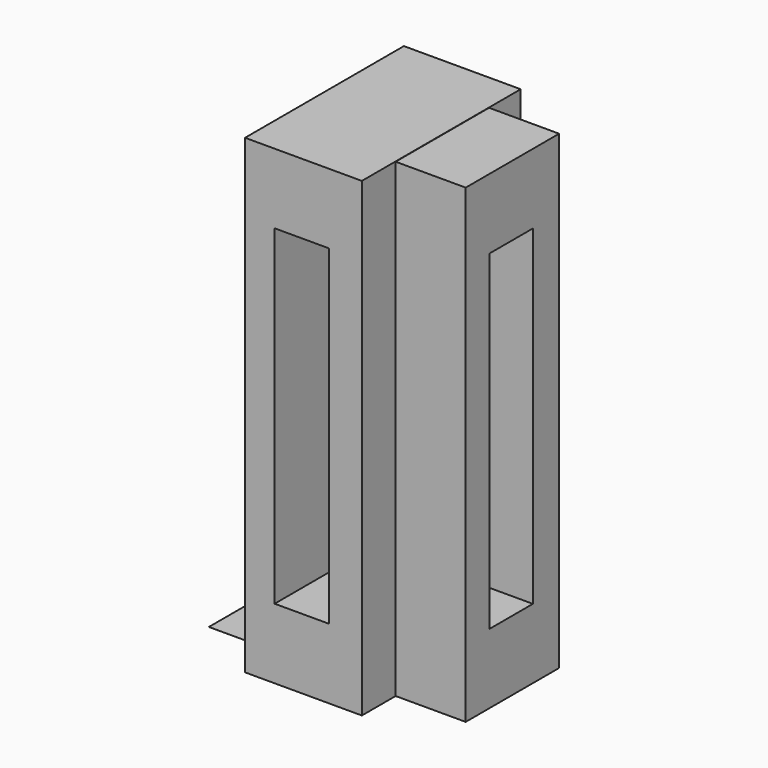
from build123d import *

# Parameters (mm, degrees)
F0_W     = 10
F0_H     = 40.3
F0_W_2   = 4.6593984449
F0_H_2   = 28.3
F1_DEPTH = 8.5
F2_DEPTH = 7
F4_W     = 10
F4_H     = 0.0023088843
F5_DEPTH = 6
F4_W_2   = 4.6593984449
F4_H_2   = 28.3
F6_DEPTH = 1
F7_W     = 10
F7_H     = 40.2760509044
F7_W_2   = 4.6593984449
F7_H_2   = 28.3
F8_DEPTH = 6
F9_DEPTH = 25.4


# Not quite as in the source:
# - a feature names something its author has since deleted; it is built from what else it names


with BuildPart() as f1:
    # F0 (on Front) → F1 (new body)
    with BuildSketch(Plane.XZ):
        with Locations((-25.2545091997, -60.7344553381)):
            Rectangle(F0_W, F0_H)
        with Locations((-25.3930282849, -60.7344553381)):
            Rectangle(F0_W_2, F0_H_2, mode=Mode.SUBTRACT)
        with Locations((-25.3930282849, -60.7344553381)):
            Rectangle(F0_W_2, F0_H_2)
    extrude(amount=F1_DEPTH)

    # F0 (on Front) → F2 (cut)
    with BuildSketch(Plane.XZ):
        with Locations((-25.3930282849, -60.7344553381)):
            Rectangle(F0_W_2, F0_H_2)
    extrude(amount=F2_DEPTH, mode=Mode.SUBTRACT)

    # F3: F1 across face


with BuildPart() as f1_1:
    add(f1.part)
    add(f1.part.mirror(Plane(origin=(-25.2545091997, -8.5, -60.7344553381), x_dir=(1, 0, 0), z_dir=(0, -1, 0))))

    # F4 (on face) → F5 (join)
    with BuildSketch(Plane(origin=(-30.2545091997, 0, 0), x_dir=(0, -1, 0), z_dir=(-1, 0, 0))):
        with Locations((8.3737515296, -80.8856097803)):
            Rectangle(F4_W, F4_H)
    extrude(amount=F5_DEPTH)

    # F4 (on face) → F6 (cut)
    with BuildSketch(Plane(origin=(-30.2545091997, 0, 0), x_dir=(0, -1, 0), z_dir=(-1, 0, 0))):
        with Locations((8.2352324444, -60.7367642224)):
            Rectangle(F4_W_2, F4_H_2)
    extrude(amount=-F6_DEPTH, mode=Mode.SUBTRACT)

    # F7 (on face) → F8 (join)
    with BuildSketch(Plane.YZ.offset(-20.2545091997)):
        with Locations((-8.3855800414, -60.7464298859)):
            Rectangle(F7_W, F7_H)
        with Locations((-8.5240991265, -60.7584044337)):
            Rectangle(F7_W_2, F7_H_2, mode=Mode.SUBTRACT)
    extrude(amount=F8_DEPTH)

    # F9 (cut): a face of the model
    f9_faces = [f1_1.faces().sort_by_distance(p)[0] for p in [
        (-20.2545091997, -8.5240991265, -60.7584044337),
    ]]
    extrude(f9_faces, amount=-F9_DEPTH, mode=Mode.SUBTRACT)


solid = f1_1.part
